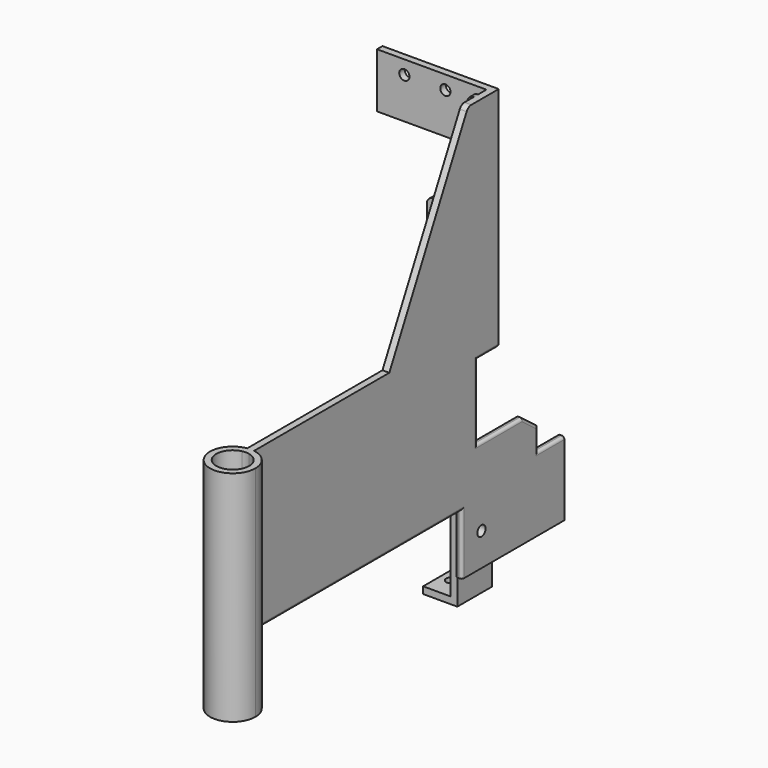
from build123d import *

# Parameters (mm, degrees)
F1_DEPTH  = 101.6
F2_W      = 120.65
F2_H      = 27.94
F3_DEPTH  = 3.175
F4_W      = 38.1
F4_H      = 15.24
F5_DEPTH  = 3.175
F7_DEPTH  = 3.175
F8_W      = 3.175
F8_H      = 25.4
F9_DEPTH  = 50.8
F10_R     = 2.38125
F11_DEPTH = 7.62
F12_W     = 2.54
F12_H     = 65.5879406387
F12_H_2   = 97.5048740911
F12_W_2   = 129.54
F12_H_3   = 2.54
F12_W_3   = 164.8392262883
F13_DEPTH = 3.048
F14_R     = 3.04799
F15_R     = 1.27
F16_W     = 20.0592262883
F16_H     = 27.94
F16_H_2   = 12.7
F17_DEPTH = 3.175
F18_R     = 2.38125
F19_DEPTH = 25.4
F21_DEPTH = 3.175
F22_W     = 20.0592262883
F22_H     = 3.175
F23_DEPTH = 12.7
F24_R     = 2.38125
F25_DEPTH = 25.4


# Not quite as in the source:
# - a fillet or chamfer is up to 0.001 mm smaller than in the source, because OpenCascade refuses the exact size


with BuildPart() as f1:
    # F0 (on Top) → F1 (new body)
    with BuildSketch(Plane.XY):
        with BuildLine():
            ThreePointArc((1.5875, 7.4528010674), (5.9228856987, 4.7941448664), (7.62, 0))
            ThreePointArc((7.62, 0), (-4.7941448664, -5.9228856987), (-1.5875, 7.4528010674))
            Line((-1.5875, 7.4528010674), (-1.5875, 10.4207737117))
            ThreePointArc((-1.5875, 10.4207737117), (-6.8694557099, -7.9952022645), (10.541, 0))
            ThreePointArc((10.541, 0), (7.9952022645, 6.8694557099), (1.5875, 10.4207737117))
            Line((1.5875, 10.4207737117), (1.5875, 7.4528010674))
        make_face()
        with BuildLine():
            ThreePointArc((-1.5875, 7.4528010674), (0, 7.62), (1.5875, 7.4528010674))
            Line((1.5875, 7.4528010674), (1.5875, 10.4207737117))
            ThreePointArc((1.5875, 10.4207737117), (0, 10.541), (-1.5875, 10.4207737117))
            Line((-1.5875, 10.4207737117), (-1.5875, 7.4528010674))
        make_face()
        with BuildLine():
            ThreePointArc((-1.5875, 10.4207737117), (0, 10.541), (1.5875, 10.4207737117))
            Line((1.5875, 10.4207737117), (1.5875, 190.5))
            Line((1.5875, 190.5), (-1.5875, 190.5))
            Line((-1.5875, 190.5), (-1.5875, 10.4207737117))
        make_face()
    extrude(amount=F1_DEPTH)

    # F2 (on face) → F3 (cut, through all)
    with BuildSketch(Plane(origin=(-1.5875, 0, 0), x_dir=(0, -1, 0), z_dir=(-1, 0, 0))):
        with Locations((-70.7457737117, 13.97)):
            Rectangle(F2_W, F2_H)
    extrude(amount=-F3_DEPTH, mode=Mode.SUBTRACT)

    # F4 (on face) → F5 (cut, through all)
    with BuildSketch(Plane(origin=(-1.5875, 0, 0), x_dir=(0, -1, 0), z_dir=(-1, 0, 0))):
        Polygon((-152.4, 86.36), (-190.5, 86.36), (-190.5, 51.562), (-175.26, 51.562), (-166.3150191307, 51.562), (-139.9607737117, 51.562), (-139.9607737117, 86.36), align=None)
        with Locations((-171.45, 93.98)):
            Rectangle(F4_W, F4_H)
        Polygon((-175.26, 51.562), (-190.5, 51.562), (-190.5, 34.29), (-175.26, 34.29), (-175.26, 44.7550229728), align=None)
        Polygon((-166.3150191307, 51.562), (-175.26, 51.562), (-175.26, 44.7550229728), align=None)
    extrude(amount=-F5_DEPTH, mode=Mode.SUBTRACT)

    # F6 (on face) → F7 (join, through all)
    with BuildSketch(Plane(origin=(-1.5875, 0, 0), x_dir=(0, -1, 0), z_dir=(-1, 0, 0))):
        Polygon((-152.4, 191.77), (-152.4, 101.6), (-88.9, 101.6), (-134.62, 191.77), align=None)
    extrude(amount=-F7_DEPTH)

    # F8 (on face) → F9 (join)
    with BuildSketch(Plane(origin=(-1.5875, 0, 0), x_dir=(0, -1, 0), z_dir=(-1, 0, 0))):
        with Locations((-150.8125, 179.07)):
            Rectangle(F8_W, F8_H)
    extrude(amount=F9_DEPTH)

    # F10 (on face) + F9_face1 (on face) → F11 (cut)
    with BuildSketch(Plane.XZ.offset(-149.225)):
        with Locations((-39.6875, 185.42)):
            Circle(F10_R)
        with Locations((-20.6375, 185.42)):
            Circle(F10_R)
    with BuildSketch(Plane(origin=(-21.429280397, 152.4, 170.8307568238), x_dir=(-1, 0, 0), z_dir=(0, 1, 0))):
        Polygon((-23.016780397, -84.4707568238), (-19.841780397, -84.4707568238), (-19.841780397, -4.4607568238), (30.958219603, -4.4607568238), (30.958219603, 20.9392431762), (-23.016780397, 20.9392431762), align=None)
    extrude(amount=-F11_DEPTH, dir=(0, -1, 0), mode=Mode.SUBTRACT)

    # F12 (on face) → F13 (join)
    with BuildSketch(Plane(origin=(-1.5875, 0, 0), x_dir=(0, -1, 0), z_dir=(-1, 0, 0))):
        with Locations((-119.7067661368, 127.0590962282)):
            Rectangle(F12_W, F12_H)
        with Locations((-143.1925, 143.0175629544)):
            Rectangle(F12_W, F12_H_2)
        Polygon((-152.4, 91.7251259089), (-10.4207737117, 91.7251259089), (-10.4207737117, 94.2651259089), (-118.4367661368, 94.2651259089), (-120.9767661368, 94.2651259089), (-141.9225, 94.2651259089), (-144.4625, 94.2651259089), (-152.4, 94.2651259089), align=None)
        with Locations((-75.1907737117, 67.31)):
            Rectangle(F12_W_2, F12_H_3)
        with Locations((-92.8403868558, 39.37)):
            Rectangle(F12_W_3, F12_H_3)
    extrude(amount=F13_DEPTH)

    # F14 (radius 3.048 in the source; OpenCascade refuses exactly that, so slightly less here)
    f14_edges = [f1.edges().sort_by_distance(p)[0] for p in [
        (0, 134.62, 191.77),
        (-4.6355, 143.1925, 191.77),
        (-4.6355, 152.4, 92.995126),
        (-4.6355, 139.960774, 67.31),
        (-4.6355, 119.706766, 159.853067),
        (-4.6355, 175.26, 39.37),
    ]]
    fillet(f14_edges, radius=F14_R)

    # F15
    f15_edges = [f1.edges().sort_by_distance(p)[0] for p in [
        (-1.5875, 170.78751, 48.158511),
        (-1.5875, 153.137896, 51.562),
        (-1.5875, 182.88, 34.29),
        (-1.5875, 175.26, 36.195),
        (-1.5875, 175.26, 42.697511),
        (1.5875, 182.88, 34.29),
        (1.5875, 175.26, 39.522511),
        (1.5875, 170.78751, 48.158511),
        (1.5875, 153.137896, 51.562),
        (-1.5875, 139.960774, 58.801),
        (-1.5875, 139.960774, 77.47),
        (1.5875, 139.960774, 68.961),
        (-1.5875, 146.180387, 86.36),
        (1.5875, 146.180387, 86.36),
        (0, 152.4, 86.36),
        (1.5875, 70.745774, 27.94),
        (-1.5875, 70.745774, 27.94),
        (1.5875, 131.070774, 13.97),
        (-1.5875, 131.070774, 13.97),
    ]]
    fillet(f15_edges, radius=F15_R)


with BuildPart() as f17:
    # F16 (on face) → F17 (new body)
    with BuildSketch(Plane(origin=(-1.5875, 0, 0), x_dir=(0, -1, 0), z_dir=(-1, 0, 0))):
        with Locations((-142.3703868558, 13.97)):
            Rectangle(F16_W, F16_H)
        with Locations((-142.3703868558, -6.35)):
            Rectangle(F16_W, F16_H_2)
    extrude(amount=F17_DEPTH)


with BuildPart() as f19_tool:
    # F18 (on face) → F19 (new body)
    with BuildSketch(Plane(origin=(-4.7625, 0, 0), x_dir=(0, -1, 0), z_dir=(-1, 0, 0))):
        with Locations((-142.3703868558, 15.24)):
            Circle(F18_R)
    extrude(amount=-F19_DEPTH)


with BuildPart() as f1_1:
    add(f1.part)

    # F19: cut by f19_tool
    add(f19_tool.part, mode=Mode.SUBTRACT)


with BuildPart() as f17_1:
    add(f17.part)

    # F19: cut by f19_tool
    add(f19_tool.part, mode=Mode.SUBTRACT)

    # F20 (on face) → F21 (cut, through all)
    with BuildSketch(Plane(origin=(-4.7625, 0, 0), x_dir=(0, -1, 0), z_dir=(-1, 0, 0))):
        with BuildLine():
            Line((-144.7490949204, 21.6999977557), (-139.9916787913, 21.6999977557))
            ThreePointArc((-139.9916787913, 21.6999977557), (-142.3703868558, 23.97125), (-144.7490949204, 21.6999977557))
        make_face()
        with BuildLine():
            Line((-139.9916787913, 21.4800022443), (-139.9916787913, 21.6999977557))
            Line((-139.9916787913, 21.6999977557), (-144.7490949204, 21.6999977557))
            Line((-144.7490949204, 21.6999977557), (-144.7490949204, 21.4800022443))
            ThreePointArc((-144.7490949204, 21.4800022443), (-142.3703868558, 19.20875), (-139.9916787913, 21.4800022443))
        make_face()
        with BuildLine():
            Line((-139.9916787913, 15.3499977557), (-139.9916787913, 21.4800022443))
            ThreePointArc((-139.9916787913, 21.4800022443), (-142.3703868558, 19.20875), (-144.7490949204, 21.4800022443))
            Line((-144.7490949204, 21.4800022443), (-144.7490949204, 15.3499977557))
            ThreePointArc((-144.7490949204, 15.3499977557), (-142.3703868558, 17.62125), (-139.9916787913, 15.3499977557))
        make_face()
        with BuildLine():
            Line((-139.9916787913, 6.9676285562), (-139.9916787913, 15.1300022443))
            ThreePointArc((-139.9916787913, 15.1300022443), (-142.3703868558, 12.85875), (-144.7490949204, 15.1300022443))
            Line((-144.7490949204, 15.1300022443), (-144.7490949204, 6.9676285562))
            ThreePointArc((-144.7490949204, 6.9676285562), (-142.3703868558, 9.2388808006), (-139.9916787913, 6.9676285562))
        make_face()
        with BuildLine():
            Line((-139.9916787913, 6.7476330449), (-139.9916787913, 6.9676285562))
            ThreePointArc((-139.9916787913, 6.9676285562), (-142.3703868558, 9.2388808006), (-144.7490949204, 6.9676285562))
            Line((-144.7490949204, 6.9676285562), (-144.7490949204, 6.7476330449))
            ThreePointArc((-144.7490949204, 6.7476330449), (-142.3703868558, 4.4763808006), (-139.9916787913, 6.7476330449))
        make_face()
    extrude(amount=-F21_DEPTH, mode=Mode.SUBTRACT)

    # F22 (on face) → F23 (join)
    with BuildSketch(Plane(origin=(-4.7625, 0, 0), x_dir=(0, -1, 0), z_dir=(-1, 0, 0))):
        with Locations((-142.3703868558, -11.1125)):
            Rectangle(F22_W, F22_H)
    extrude(amount=F23_DEPTH)

    # F24 (on face) → F25 (cut)
    with BuildSketch(Plane.XY.offset(-9.525)):
        with Locations((-12.3825, 142.3703868558)):
            Circle(F24_R)
    extrude(amount=-F25_DEPTH, mode=Mode.SUBTRACT)


solid = Compound([f1_1.part, f17_1.part])
